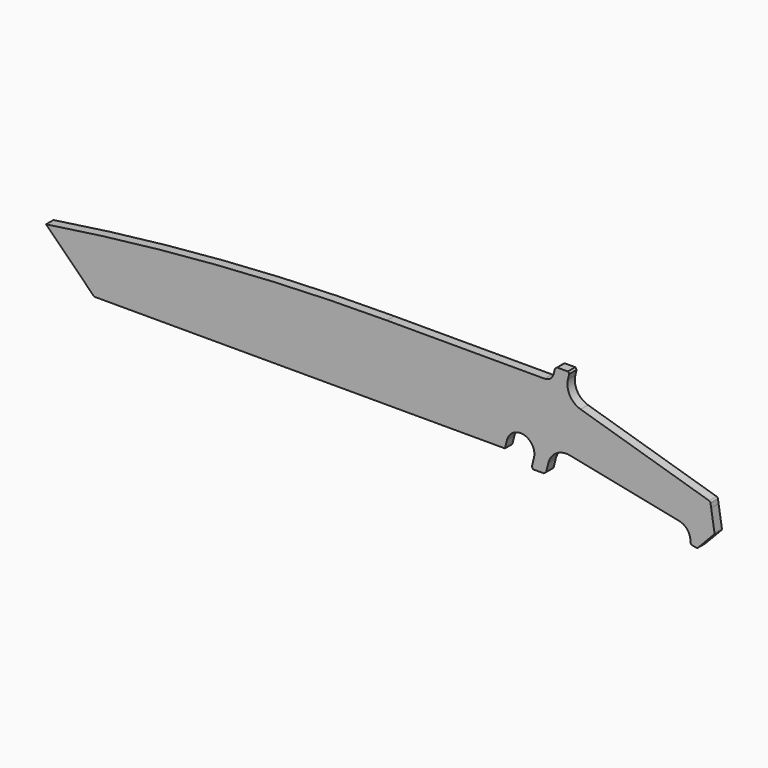
from build123d import *

# Parameters (mm, degrees)
F1_DEPTH    = 3.175
F2_SIZE2    = 1.27
F2_SIZE     = 1.27
F3_SIZE     = 1.27
F4_T1_DEPTH = 11.3354455178
F5_R        = 1.27


# Not quite as in the source:
# - a fillet or chamfer that OpenCascade refuses, or shapes differently, is made with other operations: its cross-section is extruded or revolved along the edge and cut away or added


with BuildPart() as f1:
    # F0 (on Front) → F1 (new body, symmetric)
    with BuildSketch(Plane.XZ):
        with BuildLine():
            Line((-222.2856830398, -18.875252817), (58.6383169602, -18.875252817))
            Line((58.6383169602, -18.875252817), (60.004461396, -13.3959467614))
            ThreePointArc((60.004461396, -13.3959467614), (63.3823526363, -8.1944503889), (69.2465281888, -6.175252817))
            Line((69.2465281888, -6.175252817), (-217.0251707977, -6.175252817))
            Line((-217.0251707977, -6.175252817), (-222.2856830398, -18.875252817))
        make_face()
        Polygon((-255.1717254639, 14.010789607), (-222.2856830398, -18.875252817), (-217.0251707977, -6.175252817), (-238.4935903897, 15.293166775), align=None)
        with BuildLine():
            ThreePointArc((-22.1892522704, 31.924747183), (-139.0243312187, 27.4396580434), (-255.1717254639, 14.0107896071))
            Line((-255.1717254639, 14.0107896071), (-238.4935903897, 15.293166775))
            Line((-238.4935903897, 15.293166775), (-22.1892522704, 31.924747183))
        make_face()
        with BuildLine():
            Line((-238.4935903897, 15.293166775), (-217.0251707977, -6.175252817))
            Line((-217.0251707977, -6.175252817), (69.2465281888, -6.175252817))
            ThreePointArc((69.2465281888, -6.175252817), (76.7523306169, -9.8360772646), (78.4885949816, -18.0045588726))
            Line((78.4885949816, -18.0045588726), (76.6882737813, -25.225252817))
            Line((76.6882737813, -25.225252817), (86.5048686008, -25.225252817))
            Line((86.5048686008, -25.225252817), (88.3051898011, -18.0045588726))
            ThreePointArc((88.3051898011, -18.0045588726), (93.8510411727, -10.3362236111), (103.1599182919, -8.631923198))
            Line((103.1599182919, -8.631923198), (177.815158105, -23.8207034021))
            ThreePointArc((177.815158105, -23.8207034021), (183.9152537909, -27.983372217), (185.2067697838, -35.2546145785))
            Line((185.2067697838, -35.2546145785), (190.1425618478, -36.2588128234))
            Line((190.1425618478, -36.2588128234), (192.5143319625, -33.7604418083))
            Line((192.5143319625, -33.7604418083), (199.6791825839, -8.8887735704))
            Line((199.6791825839, -8.8887735704), (199.0935677301, -5.1867834867))
            Line((199.0935677301, -5.1867834867), (110.401744257, 21.506425589))
            ThreePointArc((110.401744257, 21.506425589), (103.0219894482, 27.389702526), (101.7390811386, 36.7399899454))
            Line((101.7390811386, 36.7399899454), (102.9133555046, 41.449747183))
            Line((102.9133555046, 41.449747183), (93.096760685, 41.449747183))
            Line((93.096760685, 41.449747183), (91.9221255914, 36.7385431459))
            ThreePointArc((91.9221255914, 36.7385431459), (89.6701980979, 33.2708788976), (85.7607477296, 31.924747183))
            Line((85.7607477296, 31.924747183), (-22.1892522704, 31.924747183))
            Line((-22.1892522704, 31.924747183), (-238.4935903897, 15.293166775))
        make_face()
        Polygon((202.0282745361, -23.738661781), (199.6791825839, -8.8887735704), (192.5143319625, -33.7604418083), align=None)
    extrude(amount=F1_DEPTH, both=True)

    # F2
    f2_edges = [f1.edges().sort_by_distance(p)[0] for p in [
        (93.096761, 0, 41.449747),
        (86.504869, 0, -25.225253),
    ]]
    chamfer(f2_edges, length=F2_SIZE, length2=F2_SIZE2)

    # F3
    f3_edges = [f1.edges().sort_by_distance(p)[0] for p in [
        (102.913356, 0, 41.449747),
        (76.688274, 0, -25.225253),
    ]]
    chamfer(f3_edges, length=F3_SIZE)

    # F4: chamfer of 1.016 on 1 edges, made by hand

    # F4_s2 → F4_t1 (cut)
    with BuildSketch(Plane.XZ.offset(-5.6677227589)):
        with BuildLine():
            Line((185.3423672188, -34.3154020779), (186.1779563064, -35.4804096602))
            Line((186.1779563064, -35.4804096602), (186.1739051499, -35.5003217302))
            ThreePointArc((186.1739051499, -35.5003217302), (185.6910670267, -35.3738822533), (185.2027186274, -35.2745266485))
            Line((185.2027186274, -35.2745266485), (185.1869498558, -35.2501343047))
            ThreePointArc((185.1869498558, -35.2501343047), (185.2797978886, -34.7859194498), (185.322207486, -34.3128550063))
            Line((185.322207486, -34.3128550063), (185.3423672188, -34.3154020779))
        make_face()
    extrude(amount=F4_T1_DEPTH, mode=Mode.SUBTRACT)

    # F5
    f5_edges = [f1.edges().sort_by_distance(p)[0] for p in [
        (202.028275, 0, -23.738662),
        (199.093568, 0, -5.186783),
        (190.142562, 0, -36.258813),
    ]]
    fillet(f5_edges, radius=F5_R)


solid = f1.part
